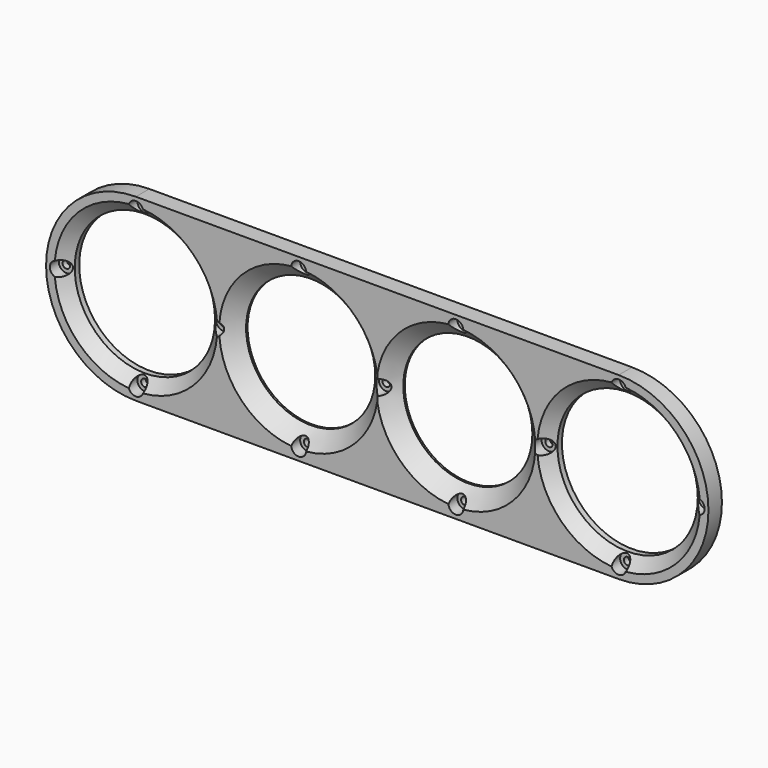
from build123d import *

# Parameters (mm, degrees)
F0_R     = 2
F0_R_2   = 37.5
F0_R_3   = 34.5
F1_DEPTH = 9
F4_R     = 4
F5_DEPTH = 6


# Not quite as in the source:
# - a fillet or chamfer that OpenCascade refuses, or shapes differently, is made with other operations: its cross-section is extruded or revolved along the edge and cut away or added


with BuildPart() as f1:
    # F0 (on Front) → F1 (new body)
    with BuildSketch(Plane.XZ):
        with BuildLine():
            ThreePointArc((129, -48), (177, 0), (129, 48))
            Line((129, 48), (0, 48))
            Line((0, 48), (-129, 48))
            ThreePointArc((-129, 48), (-177, 0), (-129, -48))
            Line((-129, -48), (0, -48))
            Line((0, -48), (129, -48))
        make_face()
        with Locations((-129, -42)):
            Circle(F0_R, mode=Mode.SUBTRACT)
        with Locations((-42, -42)):
            Circle(F0_R, mode=Mode.SUBTRACT)
        with Locations((42, -42)):
            Circle(F0_R, mode=Mode.SUBTRACT)
        with Locations((129, -42)):
            Circle(F0_R, mode=Mode.SUBTRACT)
        with Locations((-171, 0)):
            Circle(F0_R, mode=Mode.SUBTRACT)
        with Locations((-129, 0)):
            Circle(F0_R_2, mode=Mode.SUBTRACT)
        with Locations((-87, 0)):
            Circle(F0_R, mode=Mode.SUBTRACT)
        with Locations((-42, 0)):
            Circle(F0_R_3, mode=Mode.SUBTRACT)
        with Locations((-129, 42)):
            Circle(F0_R, mode=Mode.SUBTRACT)
        with Locations((-42, 42)):
            Circle(F0_R, mode=Mode.SUBTRACT)
        Circle(F0_R, mode=Mode.SUBTRACT)
        with Locations((42, 0)):
            Circle(F0_R_3, mode=Mode.SUBTRACT)
        with Locations((87, 0)):
            Circle(F0_R, mode=Mode.SUBTRACT)
        with Locations((129, 0)):
            Circle(F0_R_2, mode=Mode.SUBTRACT)
        with Locations((171, 0)):
            Circle(F0_R, mode=Mode.SUBTRACT)
        with Locations((42, 42)):
            Circle(F0_R, mode=Mode.SUBTRACT)
        with Locations((129, 42)):
            Circle(F0_R, mode=Mode.SUBTRACT)
    extrude(amount=F1_DEPTH)

    # F2: chamfer of 8 on 2 edges, made by hand

    # F2_s1 → F2_t2 (revolve, cut)
    with BuildSketch(Plane.XY):
        Polygon((84.5, -9), (76.5, -1), (76.5, -9), align=None)
    revolve(axis=Axis((42, -9, 0), (0, -1, 0)), mode=Mode.SUBTRACT)

    # F2_s3 → F2_t4 (revolve, cut)
    with BuildSketch(Plane.XY):
        Polygon((0.5, -9), (-7.5, -1), (-7.5, -9), align=None)
    revolve(axis=Axis((-42, -9, 0), (0, -1, 0)), mode=Mode.SUBTRACT)

    # F3: chamfer of 6 on 2 edges, made by hand

    # F3_s1 → F3_t2 (revolve, cut)
    with BuildSketch(Plane.XY):
        Polygon((172.5, -9), (166.5, -3), (166.5, -9), align=None)
    revolve(axis=Axis((129, -9, 0), (0, -1, 0)), mode=Mode.SUBTRACT)

    # F3_s3 → F3_t4 (revolve, cut)
    with BuildSketch(Plane.XY):
        Polygon((-85.5, -9), (-91.5, -3), (-91.5, -9), align=None)
    revolve(axis=Axis((-129, -9, 0), (0, -1, 0)), mode=Mode.SUBTRACT)

    # F4 (on face) → F5 (cut)
    with BuildSketch(Plane.XZ.offset(9)):
        Circle(F4_R)
        with Locations((42, 42)):
            Circle(F4_R)
        with Locations((42, -42)):
            Circle(F4_R)
        with Locations((129, 42)):
            Circle(F4_R)
        with Locations((87, 0)):
            Circle(F4_R)
        with Locations((129, -42)):
            Circle(F4_R)
        with Locations((171, 0)):
            Circle(F4_R)
        with Locations((-42, 42)):
            Circle(F4_R)
        with Locations((-42, -42)):
            Circle(F4_R)
        with Locations((-87, 0)):
            Circle(F4_R)
        with Locations((-129, -42)):
            Circle(F4_R)
        with Locations((-129, 42)):
            Circle(F4_R)
        with Locations((-171, 0)):
            Circle(F4_R)
    extrude(amount=-F5_DEPTH, mode=Mode.SUBTRACT)


solid = f1.part
